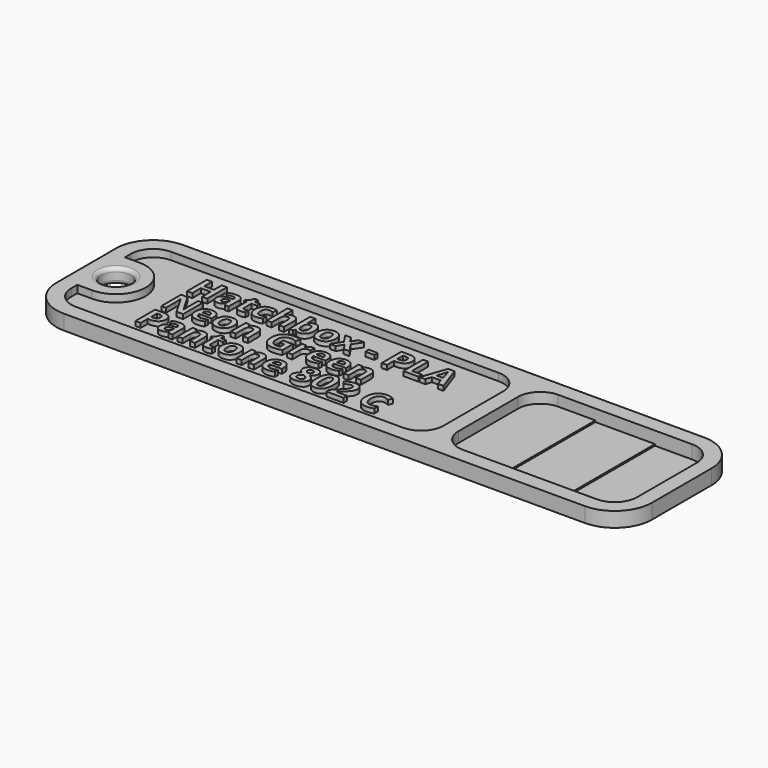
from build123d import *

# Parameters (mm, degrees)
F1_DEPTH      = 2
F3_DEPTH      = 1
F4_R          = 2
F5_DEPTH      = 2.001
F6_R          = 0.5
F7_DEPTH      = 0.4
F9_DEPTH      = 0.2
F11_DEPTH     = 0.2
F12_TEXT_SIZE = 4.6296296296
F13_DEPTH     = 0.6


# Not quite as in the source:
# - Text() gives the source's letters only with a copy of the font that has no kerning and outlines rounded to 1/6400 em; it was checked with that copy


with BuildPart() as f1:
    # F0 (on Top) → F1 (new body)
    with BuildSketch(Plane.XY):
        with BuildLine():
            ThreePointArc((40, 5), (38.5355339059, 8.5355339059), (35, 10))
            Line((35, 10), (-35, 10))
            ThreePointArc((-35, 10), (-38.5355339059, 8.5355339059), (-40, 5))
            Line((-40, 5), (-40, -5))
            ThreePointArc((-40, -5), (-38.5355339059, -8.5355339059), (-35, -10))
            Line((-35, -10), (35, -10))
            ThreePointArc((35, -10), (38.5355339059, -8.5355339059), (40, -5))
            Line((40, -5), (40, 5))
        make_face()
    extrude(amount=F1_DEPTH)

    # F2 (on face) → F3 (cut)
    with BuildSketch(Plane.XY.offset(2)):
        with BuildLine():
            ThreePointArc((35, -8), (37.1213203436, -7.1213203436), (38, -5))
            Line((38, -5), (38, 5))
            ThreePointArc((38, 5), (37.1213203436, 7.1213203436), (35, 8))
            Line((35, 8), (17, 8))
            ThreePointArc((17, 8), (14.8786796564, 7.1213203436), (14, 5))
            Line((14, 5), (14, -5))
            ThreePointArc((14, -5), (14.8786796564, -7.1213203436), (17, -8))
            Line((17, -8), (35, -8))
        make_face()
        with BuildLine():
            ThreePointArc((-38, -5), (-37.1213203436, -7.1213203436), (-35, -8))
            Line((-35, -8), (9, -8))
            ThreePointArc((9, -8), (11.1213203436, -7.1213203436), (12, -5))
            Line((12, -5), (12, 5))
            ThreePointArc((12, 5), (11.1213203436, 7.1213203436), (9, 8))
            Line((9, 8), (-35, 8))
            ThreePointArc((-35, 8), (-37.1213203436, 7.1213203436), (-38, 5))
            Line((-38, 5), (-38, 4))
            Line((-38, 4), (-36, 4))
            ThreePointArc((-36, 4), (-32, 0), (-36, -4))
            Line((-36, -4), (-38, -4))
            Line((-38, -4), (-38, -5))
        make_face()
    extrude(amount=-F3_DEPTH, mode=Mode.SUBTRACT)

    # F4 (on face) → F5 (cut, through all)
    with BuildSketch(Plane.XY.offset(2)):
        with Locations((-36, 0)):
            Circle(F4_R)
    extrude(amount=-F5_DEPTH, mode=Mode.SUBTRACT)

    # F6
    f6_edges = [f1.edges().sort_by_distance(p)[0] for p in [
        (-38, 0, 2),
        (-38, 0, 0),
    ]]
    fillet(f6_edges, radius=F6_R)

    # F7 (cut): a face of the model
    f7_faces = [f1.faces().sort_by_distance(p)[0] for p in [
        (26, 0, 1),
    ]]
    extrude(f7_faces, amount=-F7_DEPTH, mode=Mode.SUBTRACT)

    # F8 (on face) → F9 (cut)
    with BuildSketch(Plane.XY.offset(0.6)):
        with BuildLine():
            Line((22, -8), (35, -8))
            ThreePointArc((35, -8), (37.1213203436, -7.1213203436), (38, -5))
            Line((38, -5), (38, 5))
            ThreePointArc((38, 5), (37.1213203436, 7.1213203436), (35, 8))
            Line((35, 8), (22, 8))
            Line((22, 8), (22, -8))
        make_face()
    extrude(amount=-F9_DEPTH, mode=Mode.SUBTRACT)

    # F10 (on face) → F11 (cut)
    with BuildSketch(Plane.XY.offset(0.4)):
        with BuildLine():
            ThreePointArc((38, 5), (37.1213203436, 7.1213203436), (35, 8))
            Line((35, 8), (30, 8))
            Line((30, 8), (30, -8))
            Line((30, -8), (35, -8))
            ThreePointArc((35, -8), (37.1213203436, -7.1213203436), (38, -5))
            Line((38, -5), (38, 5))
        make_face()
    extrude(amount=-F11_DEPTH, mode=Mode.SUBTRACT)

    # F12 (on face) → F13 (join)
    with BuildSketch(Plane.XY.offset(1)):
        with Locations((-29, 2.6666666667)):
            Text('Hatchbox - PLA', F12_TEXT_SIZE, font='Open Sans', font_style=FontStyle.BOLD, text_align=(TextAlign.LEFT, TextAlign.BOTTOM))
        with Locations((-29, -1.6666666667)):
            Text('Neon Green', F12_TEXT_SIZE, font='Open Sans', font_style=FontStyle.BOLD, text_align=(TextAlign.LEFT, TextAlign.BOTTOM))
        with Locations((-29, -6)):
            Text('Pantone 802 C', F12_TEXT_SIZE, font='Open Sans', font_style=FontStyle.BOLD, text_align=(TextAlign.LEFT, TextAlign.BOTTOM))
    extrude(amount=F13_DEPTH)


solid = f1.part
